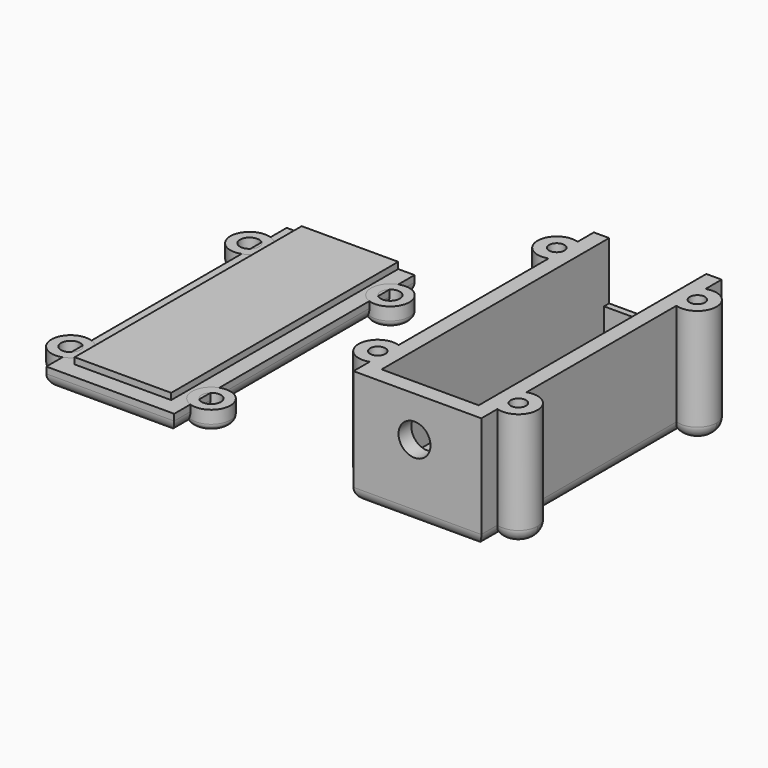
from build123d import *
from build123d import SkipClean  # not in build123d's __all__

# Parameters (mm, degrees)
F0_W           = 20
F0_H           = 47
F1_DEPTH       = 18
F2_R           = 2
F3_W           = 15.2
F3_H           = 44.5
F4_DEPTH       = 14
F8_W           = 15.2
F8_H           = 1
F9_DEPTH       = 5
F10_R          = 2.5
F11_DEPTH      = 10
F12_W          = 20
F12_H          = 47
F13_DEPTH      = 3
F14_W          = 15.1
F14_H          = 44.4
F15_DEPTH      = 1
F17_R          = 3
F19_DEPTH      = 18
F18_R          = 3
F20_DEPTH      = 3
F21_S5_R       = 2
F21_T6_DEPTH   = 6
F21_T10_ANGLE  = 180
F21_S11_R      = 2
F21_T12_DEPTH  = 5
F21_T16_ANGLE  = 180
F21_S17_R      = 2
F21_T18_DEPTH  = 5
F21_T22_ANGLE  = 180
F21_S23_R      = 2
F21_T24_DEPTH  = 5
F21_T28_ANGLE  = 180
F21_S29_R      = 2
F21_T30_DEPTH  = 5
F21_S35_R      = 2
F21_T36_DEPTH  = 6
F21_2_T1_DEPTH = 57
F21_2_T3_DEPTH = 30
F22_R          = 1
F22_2_R        = 1
F22_3_R        = 1
F22_4_R        = 1
F24_R          = 1.2
F25_DEPTH      = 14
F23_R          = 1.5
F26_DEPTH      = 5


# Not quite as in the source:
# - a fillet or chamfer that OpenCascade refuses, or shapes differently, is made with other operations: its cross-section is extruded or revolved along the edge and cut away or added
# - a feature of the source that left no trace in its solid (it failed there, or was rolled back) is left out
# - the program builds the solid bodies; features that only make, move or delete a surface that nothing else refers to are left out


with BuildPart() as f1:
    # F0 (on Top) → F1 (new body)
    with BuildSketch(Plane.XY):
        Rectangle(F0_W, F0_H)
    extrude(amount=F1_DEPTH)

    # F2
    f2_edges = [f1.edges().sort_by_distance(p)[0] for p in [
        (-10, 0, 0),
        (0, 23.5, 0),
        (10, 0, 0),
        (0, -23.5, 0),
    ]]
    fillet(f2_edges, radius=F2_R)

    # F3 (on face) → F4 (cut)
    with BuildSketch(Plane.XY.offset(18)):
        with Locations((0, 1.25)):
            Rectangle(F3_W, F3_H)
    extrude(amount=-F4_DEPTH, mode=Mode.SUBTRACT)

    # F8 (on face) → F9 (join)
    with BuildSketch(Plane.XY.offset(4)):
        with Locations((0, 23)):
            Rectangle(F8_W, F8_H)
    extrude(amount=F9_DEPTH)

    # F10 (on face) → F11 (cut)
    with BuildSketch(Plane.XZ.offset(23.5)):
        with Locations((-0.4522884265, 11.6613497958)):
            Circle(F10_R)
    extrude(amount=-F11_DEPTH, mode=Mode.SUBTRACT)

    # F17 (on Top) → F19 (join)
    with BuildSketch(Plane.XY):
        with Locations((11, 17.5)):
            Circle(F17_R)
        with Locations((11, -17.5)):
            Circle(F17_R)
        with Locations((-11, 17.5)):
            Circle(F17_R)
        with Locations((-11, -17.5)):
            Circle(F17_R)
    with SkipClean():  # cleaning this boolean's faces spoils the solid; the shape is the same uncleaned
        extrude(amount=F19_DEPTH)

    # F21: fillet of radius 2 on 6 edges, made by hand


with BuildPart() as f13:
    # F12 (on Top) → F13 (new body)
    with BuildSketch(Plane.XY):
        with Locations((-48.0490680784, 0)):
            Rectangle(F12_W, F12_H)
    extrude(amount=F13_DEPTH)

    # F14 (on face) → F15 (join)
    with BuildSketch(Plane.XY.offset(3)):
        with Locations((-48.1490680784, 1.3)):
            Rectangle(F14_W, F14_H)
    extrude(amount=F15_DEPTH)

    # F21#2: fillet of radius 2 on 4 edges, made by hand

    # F21_2_s2 → F21_2_t1 (cut)
    with BuildSketch(Plane.XZ.offset(-28.5)):
        with BuildLine():
            ThreePointArc((-38.0490680784, 2), (-38.634854516, 0.5857864376), (-40.0490680784, 0))
            Line((-40.0490680784, 0), (-38.0490680784, 0))
            Line((-38.0490680784, 0), (-38.0490680784, 2))
        make_face()
        with BuildLine():
            ThreePointArc((-56.0490680784, 0), (-57.4632816408, 0.5857864376), (-58.0490680784, 2))
            Line((-58.0490680784, 2), (-58.0490680784, 0))
            Line((-58.0490680784, 0), (-56.0490680784, 0))
        make_face()
    extrude(amount=F21_2_T1_DEPTH, mode=Mode.SUBTRACT)

    # F21_2_s4 → F21_2_t3 (cut)
    with BuildSketch(Plane.YZ.offset(-63.0490680784)):
        with BuildLine():
            ThreePointArc((-23.5, 2), (-22.9142135624, 0.5857864376), (-21.5, 0))
            Line((-21.5, 0), (-23.5, 0))
            Line((-23.5, 0), (-23.5, 2))
        make_face()
        with BuildLine():
            ThreePointArc((23.5, 2), (22.9142135624, 0.5857864376), (21.5, 0))
            Line((21.5, 0), (23.5, 0))
            Line((23.5, 0), (23.5, 2))
        make_face()
    extrude(amount=F21_2_T3_DEPTH, mode=Mode.SUBTRACT)


with BuildPart() as f20:
    # F18 (on Top) → F20 (new body)
    with BuildSketch(Plane.XY):
        with Locations((-37.0490680784, 17.5)):
            Circle(F18_R)
    extrude(amount=F20_DEPTH)

    # F22
    f22_edges = [f20.edges().sort_by_distance(p)[0] for p in [
        (-40.049068, 17.5, 0),
    ]]
    fillet(f22_edges, radius=F22_R)


with BuildPart() as f20b:
    # F18 (on Top) → F20, piece 2 (new body)
    with BuildSketch(Plane.XY):
        with Locations((-37.0490680784, -17.5)):
            Circle(F18_R)
    extrude(amount=F20_DEPTH)

    # F22#2
    f22_2_edges = [f20b.edges().sort_by_distance(p)[0] for p in [
        (-40.049068, -17.5, 0),
    ]]
    fillet(f22_2_edges, radius=F22_2_R)


with BuildPart() as f20c:
    # F18 (on Top) → F20, piece 3 (new body)
    with BuildSketch(Plane.XY):
        with Locations((-59.0490680784, 17.5)):
            Circle(F18_R)
    extrude(amount=F20_DEPTH)

    # F22#3
    f22_3_edges = [f20c.edges().sort_by_distance(p)[0] for p in [
        (-62.049068, 17.5, 0),
    ]]
    fillet(f22_3_edges, radius=F22_3_R)


with BuildPart() as f20d:
    # F18 (on Top) → F20, piece 4 (new body)
    with BuildSketch(Plane.XY):
        with Locations((-59.0490680784, -17.5)):
            Circle(F18_R)
    extrude(amount=F20_DEPTH)

    # F22#4
    f22_4_edges = [f20d.edges().sort_by_distance(p)[0] for p in [
        (-62.049068, -17.5, 0),
    ]]
    fillet(f22_4_edges, radius=F22_4_R)


with BuildPart() as f21_tool2:
    # F21_s3 → F21_t4 (revolve)
    with BuildSketch(Plane.XZ.offset(-17.5)):
        with BuildLine():
            ThreePointArc((-8, 2), (-8.5857864376, 0.5857864376), (-10, 0))
            Line((-10, 0), (-8, 0))
            Line((-8, 0), (-8, 2))
        make_face()
    revolve(axis=Axis((-11, 17.5, 0), (0, 0, 1)))

    # F21_s5 → F21_t6 (cut, symmetric)
    with BuildSketch(Plane.XZ.offset(-17.5)):
        with Locations((-8, 2)):
            Circle(F21_S5_R)
    extrude(amount=F21_T6_DEPTH, both=True, mode=Mode.SUBTRACT)


with BuildPart() as f1_1:
    add(f1.part, clean=False)

    # F21_t1: cut F21_tool2
    add(f21_tool2.part, mode=Mode.SUBTRACT)


with BuildPart() as f21_tool8:
    # F21_s9 → F21_t10 (revolve)
    with BuildSketch(Plane.XZ.offset(-17.5)):
        with BuildLine():
            ThreePointArc((14, 2), (13.4142135624, 0.5857864376), (12, 0))
            Line((12, 0), (14, 0))
            Line((14, 0), (14, 2))
        make_face()
    revolve(axis=Axis((11, 17.5, 0), (0, 0, 1)), revolution_arc=F21_T10_ANGLE)

    # F21_s11 → F21_t12 (cut, symmetric)
    with BuildSketch(Plane.XZ.offset(-19)):
        with Locations((8, 2)):
            Circle(F21_S11_R)
    extrude(amount=F21_T12_DEPTH, both=True, mode=Mode.SUBTRACT)


with BuildPart() as f1_2:
    add(f1_1.part, clean=False)

    # F21_t7: cut F21_tool8
    add(f21_tool8.part, mode=Mode.SUBTRACT)


with BuildPart() as f21_tool14:
    # F21_s15 → F21_t16 (revolve)
    with BuildSketch(Plane.XZ.offset(-17.5)):
        with BuildLine():
            ThreePointArc((10, 0), (8.5857864376, 0.5857864376), (8, 2))
            Line((8, 2), (8, 0))
            Line((8, 0), (10, 0))
        make_face()
    revolve(axis=Axis((11, 17.5, 0), (0, 0, 1)), revolution_arc=F21_T16_ANGLE)

    # F21_s17 → F21_t18 (cut, symmetric)
    with BuildSketch(Plane.XZ.offset(-16)):
        with Locations((8, 2)):
            Circle(F21_S17_R)
    extrude(amount=F21_T18_DEPTH, both=True, mode=Mode.SUBTRACT)


with BuildPart() as f1_3:
    add(f1_2.part, clean=False)

    # F21_t13: cut F21_tool14
    add(f21_tool14.part, mode=Mode.SUBTRACT)


with BuildPart() as f21_tool20:
    # F21_s21 → F21_t22 (revolve)
    with BuildSketch(Plane.XZ.offset(17.5)):
        with BuildLine():
            ThreePointArc((14, 2), (13.4142135624, 0.5857864376), (12, 0))
            Line((12, 0), (14, 0))
            Line((14, 0), (14, 2))
        make_face()
    revolve(axis=Axis((11, -17.5, 0), (0, 0, 1)), revolution_arc=F21_T22_ANGLE)

    # F21_s23 → F21_t24 (cut, symmetric)
    with BuildSketch(Plane.XZ.offset(16)):
        with Locations((8, 2)):
            Circle(F21_S23_R)
    extrude(amount=F21_T24_DEPTH, both=True, mode=Mode.SUBTRACT)


with BuildPart() as f1_4:
    add(f1_3.part, clean=False)

    # F21_t19: cut F21_tool20
    add(f21_tool20.part, mode=Mode.SUBTRACT)


with BuildPart() as f21_tool26:
    # F21_s27 → F21_t28 (revolve)
    with BuildSketch(Plane.XZ.offset(17.5)):
        with BuildLine():
            ThreePointArc((8, 2), (8.5857864376, 0.5857864376), (10, 0))
            Line((10, 0), (8, 0))
            Line((8, 0), (8, 2))
        make_face()
    revolve(axis=Axis((11, -17.5, 0), (0, 0, 1)), revolution_arc=F21_T28_ANGLE)

    # F21_s29 → F21_t30 (cut, symmetric)
    with BuildSketch(Plane.XZ.offset(19)):
        with Locations((8, 2)):
            Circle(F21_S29_R)
    extrude(amount=F21_T30_DEPTH, both=True, mode=Mode.SUBTRACT)


with BuildPart() as f1_5:
    add(f1_4.part, clean=False)

    # F21_t25: cut F21_tool26
    add(f21_tool26.part, mode=Mode.SUBTRACT)


with BuildPart() as f21_tool32:
    # F21_s33 → F21_t34 (revolve)
    with BuildSketch(Plane.XZ.offset(17.5)):
        with BuildLine():
            ThreePointArc((-8, 2), (-8.5857864376, 0.5857864376), (-10, 0))
            Line((-10, 0), (-8, 0))
            Line((-8, 0), (-8, 2))
        make_face()
    revolve(axis=Axis((-11, -17.5, 0), (0, 0, 1)))

    # F21_s35 → F21_t36 (cut, symmetric)
    with BuildSketch(Plane.XZ.offset(17.5)):
        with Locations((-8, 2)):
            Circle(F21_S35_R)
    extrude(amount=F21_T36_DEPTH, both=True, mode=Mode.SUBTRACT)


with BuildPart() as f1_6:
    add(f1_5.part, clean=False)

    # F21_t31: cut F21_tool32
    add(f21_tool32.part, mode=Mode.SUBTRACT)

    # F24 (on face) → F25 (cut)
    with BuildSketch(Plane.XY.offset(18)):
        with Locations((11, 17.5)):
            Circle(F24_R)
        with Locations((11, -17.5)):
            Circle(F24_R)
        with Locations((-11, 17.5)):
            Circle(F24_R)
        with Locations((-11, -17.5)):
            Circle(F24_R)
    extrude(amount=-F25_DEPTH, mode=Mode.SUBTRACT)


with BuildPart() as f26_tool:
    # F23 (on face) → F26 (new body)
    with BuildSketch(Plane.XY.offset(3)):
        with Locations((-37.0490680784, 17.5)):
            Circle(F23_R)
        with Locations((-59.0490680784, 17.5)):
            Circle(F23_R)
        with Locations((-59.0490680784, -17.5)):
            Circle(F23_R)
        with Locations((-37.0490680784, -17.5)):
            Circle(F23_R)
    extrude(amount=-F26_DEPTH)


with BuildPart() as f20_1:
    add(f20.part, clean=False)

    # F26: cut by f26_tool
    add(f26_tool.part, mode=Mode.SUBTRACT)


with BuildPart() as f20b_1:
    add(f20b.part, clean=False)

    # F26: cut by f26_tool
    add(f26_tool.part, mode=Mode.SUBTRACT)


with BuildPart() as f20c_1:
    add(f20c.part, clean=False)

    # F26: cut by f26_tool
    add(f26_tool.part, mode=Mode.SUBTRACT)


with BuildPart() as f20d_1:
    add(f20d.part, clean=False)

    # F26: cut by f26_tool
    add(f26_tool.part, mode=Mode.SUBTRACT)


solid = Compound([f13.part, f1_6.part, f20_1.part, f20b_1.part, f20c_1.part, f20d_1.part])
